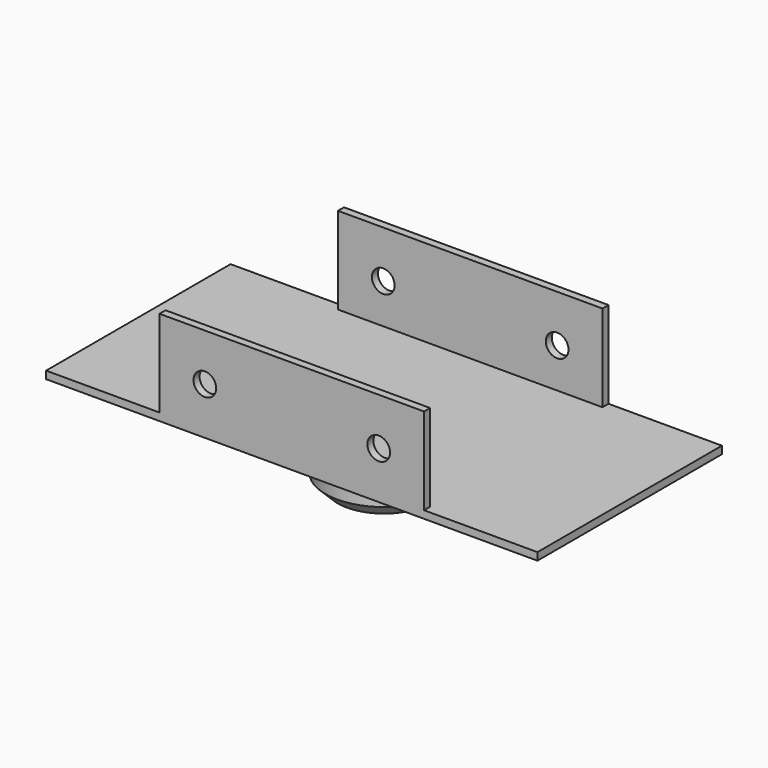
from build123d import *

# Parameters (mm, degrees)
F0_R      = 15.45
F0_R_2    = 12.25
F1_DEPTH  = 20
F2_W      = 70
F2_H      = 57
F3_DEPTH  = 2
F4_W      = 70
F4_H      = 25
F5_DEPTH  = 2
F6_W      = 70
F6_H      = 25
F7_DEPTH  = 2
F10_D     = 6
F11_W     = 61
F11_H     = 2
F12_DEPTH = 30
F14_DEPTH = 30


# Not quite as in the source:
# - a fillet or chamfer that OpenCascade refuses, or shapes differently, is made with other operations: its cross-section is extruded or revolved along the edge and cut away or added


with BuildPart() as f1:
    # F0 (on Top) → F1 (new body)
    with BuildSketch(Plane.XY):
        Circle(F0_R)
        Circle(F0_R_2, mode=Mode.SUBTRACT)
    extrude(amount=F1_DEPTH)

    # F2 (on face) → F3 (join)
    with BuildSketch(Plane.XY.offset(20)):
        Rectangle(F2_W, F2_H)
    extrude(amount=F3_DEPTH)

    # F4 (on face) → F5 (join)
    with BuildSketch(Plane.XZ.offset(28.5)):
        with Locations((0, 32.5)):
            Rectangle(F4_W, F4_H)
    extrude(amount=F5_DEPTH)

    # F6 (on face) → F7 (join)
    with BuildSketch(Plane(origin=(0, 28.5, 0), x_dir=(-1, 0, 0), z_dir=(0, 1, 0))):
        with Locations((0, 32.5)):
            Rectangle(F6_W, F6_H)
    extrude(amount=F7_DEPTH)

    # F8: chamfer of 7 on 3 edges, made by hand

    # F8_s1 → F8_t2 (revolve)
    with BuildSketch(Plane.XZ):
        Polygon((22.45, 20), (15.45, 13), (15.45, 20), align=None)
    revolve(axis=Axis((0, 0, 20), (0, 0, 1)))

    # F8_s3 → F8_t4 (revolve, cut)
    with BuildSketch(Plane.XZ):
        Polygon((15.45, 7), (8.45, 0), (15.45, 0), align=None)
    revolve(axis=Axis((0, 0, 0), (0, 0, 1)), mode=Mode.SUBTRACT)

    # F10 (through all)
    with Locations(Plane.XZ.offset(30.5)):
        with Locations((-23, 32.5), (23, 32.5)):
            Hole(F10_D / 2)

    # F11 (on face) → F12 (join)
    with BuildSketch(Plane(origin=(-35, 0, 0), x_dir=(0, -1, 0), z_dir=(-1, 0, 0))):
        with Locations((0, 21)):
            Rectangle(F11_W, F11_H)
    extrude(amount=F12_DEPTH)

    # F13 (on face) → F14 (join)
    with BuildSketch(Plane.YZ.offset(35)):
        Polygon((-30.5, 22), (-30.5, 20), (30.5, 20), (30.5, 22), (28.5, 22), (-28.5, 22), align=None)
    extrude(amount=F14_DEPTH)


solid = f1.part
